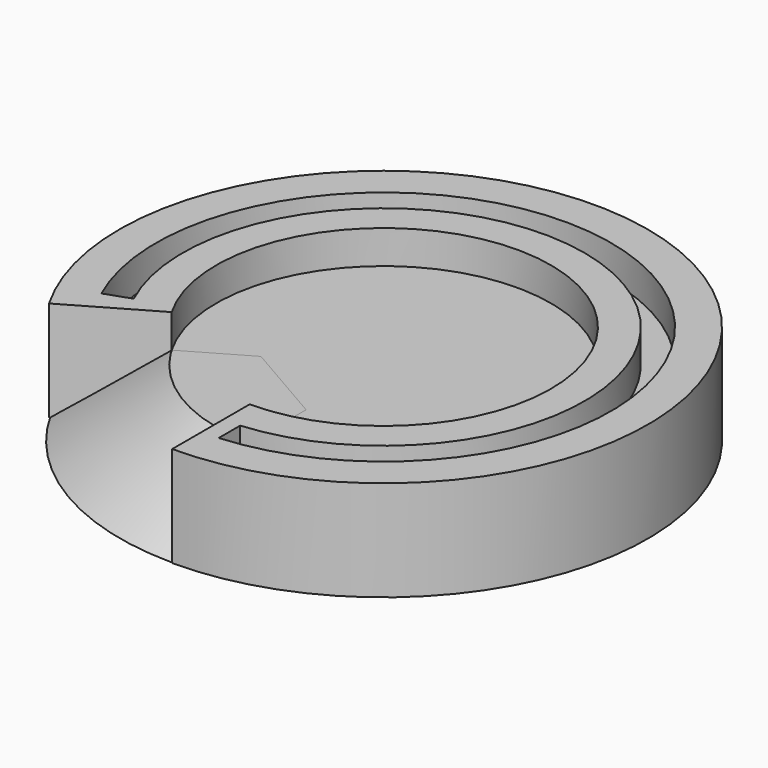
from build123d import *

# Parameters (mm, degrees)
F2_R     = 78.9342131776
F3_DEPTH = 30
F5_DEPTH = 30
F7_DEPTH = 10
F8_DEPTH = 10


with BuildPart() as f1:
    # F0 (on Right) → F1 (revolve)
    with BuildSketch(Plane.YZ):
        Polygon((-117.4011141722, 6.0772849967), (-117.4011141722, 26.0772849967), (-167.4011141722, 26.0772849967), (-196.1239274049, 6.0772849967), align=None)
    revolve(axis=Axis((0, -117.4011141722, 16.0772849967), (0, 0, -1)))


with BuildPart() as f3:
    # F2 (on face) → F3 (new body)
    with BuildSketch(Plane(origin=(0, 0, 6.0772849967), x_dir=(1, 0, 0), z_dir=(0, 0, -1))):
        with Locations((0, 117.4011141722)):
            Circle(F2_R)
    extrude(amount=-F3_DEPTH)

    # F4 (on face) → F5 (cut)
    with BuildSketch(Plane(origin=(0, 0, 6.0772849967), x_dir=(1, 0, 0), z_dir=(0, 0, -1))):
        with BuildLine():
            ThreePointArc((0, 196.3353273498), (-39.4671065888, 185.7601480117), (-68.3590338395, 156.868220761))
            Line((-68.3590338395, 156.868220761), (-25.0577636503, 131.868220761))
            Line((-25.0577636503, 131.868220761), (0, 146.3353273498))
            Line((0, 146.3353273498), (0, 196.3353273498))
        make_face()
    extrude(amount=-F5_DEPTH, mode=Mode.SUBTRACT)

    # F6 (on face) → F7 (cut)
    with BuildSketch(Plane.XY.offset(36.0772849967)):
        with BuildLine():
            ThreePointArc((4.9891766792, -185.1979539584), (49.8019499741, -163.6728025756), (67.9801689386, -117.4011141722))
            ThreePointArc((67.9801689386, -117.4011141722), (-14.2643778849, -50.9343488494), (-61.9939385535, -145.2947505711))
            Line((-61.9939385535, -145.2947505711), (-54.4301717399, -142.6470327407))
            ThreePointArc((-54.4301717399, -142.6470327407), (-12.9265172341, -58.8101152714), (60, -117.4011141722))
            ThreePointArc((60, -117.4011141722), (44.1551276793, -158.0253027749), (4.9891766792, -177.1933219928))
            Line((4.9891766792, -177.1933219928), (4.9891766792, -185.1979539584))
        make_face()
    extrude(amount=-F7_DEPTH, mode=Mode.SUBTRACT)

    # F6 (on face) → F8 (cut)
    with BuildSketch(Plane.XY.offset(36.0772849967)):
        with BuildLine():
            Line((-25.0577636503, -131.868220761), (-43.3012701892, -142.4011141722))
            ThreePointArc((-43.3012701892, -142.4011141722), (-25, -160.7023843614), (0, -167.4011141722))
            Line((0, -167.4011141722), (0, -146.3353273498))
            Line((0, -146.3353273498), (-25.0577636503, -131.868220761))
        make_face()
        with BuildLine():
            ThreePointArc((50, -117.4011141722), (-12.9409522551, -69.1048228578), (-43.3012701892, -142.4011141722))
            Line((-43.3012701892, -142.4011141722), (-25.0577636503, -131.868220761))
            Line((-25.0577636503, -131.868220761), (0, -146.3353273498))
            Line((0, -146.3353273498), (0, -167.4011141722))
            ThreePointArc((0, -167.4011141722), (35.3553390593, -152.7564532316), (50, -117.4011141722))
        make_face()
    extrude(amount=-F8_DEPTH, mode=Mode.SUBTRACT)


solid = Compound([f1.part, f3.part])
